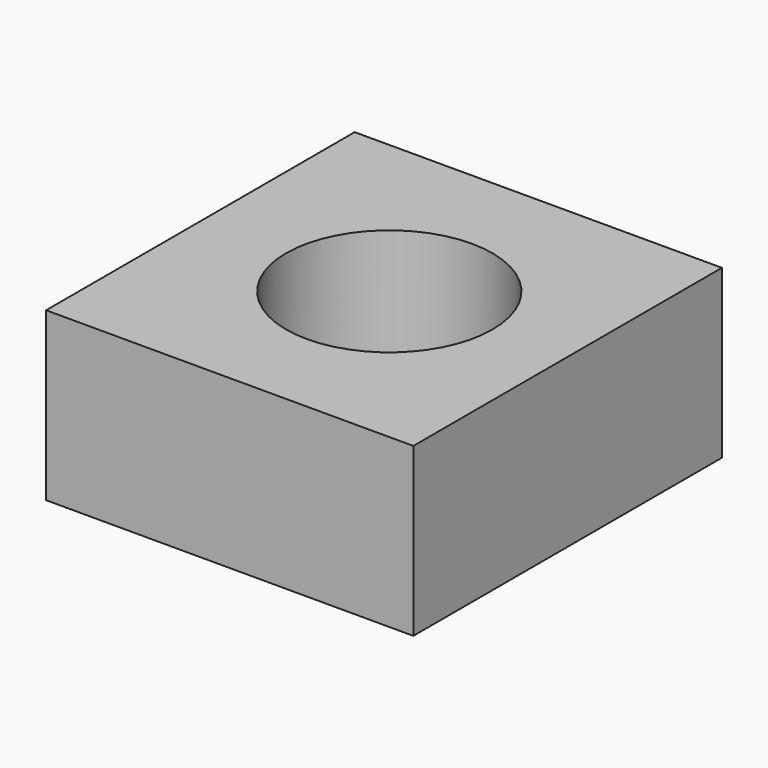
from build123d import *

# Parameters (mm, degrees)
F0_W     = 55.7806007564
F0_H     = 58.5907548666
F0_R     = 15.6812666629
F1_DEPTH = 25.4


# Not quite as in the source:
# - a feature names something its author has since deleted; it is built from what else it names


with BuildPart() as f1:
    # F0 (on Top) → F1 (new body)
    with BuildSketch(Plane.XY):
        with Locations((-0.8635763079, 0.0774934888)):
            Rectangle(F0_W, F0_H)
        Circle(F0_R, mode=Mode.SUBTRACT)
    extrude(amount=F1_DEPTH)


solid = f1.part
